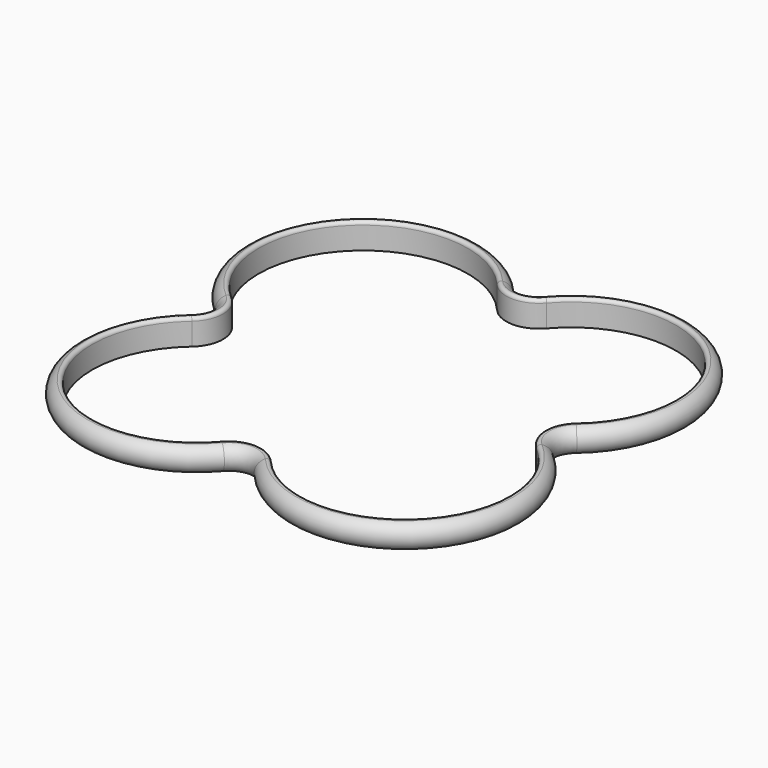
from build123d import *

# Parameters (mm, degrees)
F3_T3_ANGLE  = 98.5086767383
F3_T6_ANGLE  = 188.5086767383
F3_T9_ANGLE  = 98.5086767383
F3_T12_ANGLE = 188.5086767383
F3_T15_ANGLE = 98.5086767383
F3_T18_ANGLE = 188.5086767383
F3_T21_ANGLE = 98.5086767383
F3_T24_ANGLE = 188.5086767383


# Not quite as in the source:
# - a fillet or chamfer that OpenCascade refuses, or shapes differently, is made with other operations: its cross-section is extruded or revolved along the edge and cut away or added


with BuildPart() as f2:
    # F2: sweep along a path in F0
    with BuildLine(Plane.XY) as f2_path:
        ThreePointArc((-7.5761430926, 52.7062817331), (-54.4472211271, 54.4472231756), (-52.706281448, 7.5761450757))
        ThreePointArc((-52.706281448, 7.5761450757), (-49.2333054771, 9.262e-07), (-52.7062817331, -7.5761430926))
        ThreePointArc((-52.7062817331, -7.5761430926), (-54.4472231756, -54.4472211271), (-7.5761450757, -52.706281448))
        ThreePointArc((-7.5761450757, -52.706281448), (-9.262e-07, -49.2333054771), (7.5761430926, -52.7062817331))
        ThreePointArc((7.5761430926, -52.7062817331), (54.4472211271, -54.4472231756), (52.706281448, -7.5761450757))
        ThreePointArc((52.706281448, -7.5761450757), (49.2333054771, -9.262e-07), (52.7062817331, 7.5761430926))
        ThreePointArc((52.7062817331, 7.5761430926), (54.4472231756, 54.4472211271), (7.5761450757, 52.706281448))
        ThreePointArc((7.5761450757, 52.706281448), (9.262e-07, 49.2333054771), (-7.5761430926, 52.7062817331))
    # F1 (on Front) → F2 (sweep)
    with BuildSketch(Plane.XZ):
        with BuildLine():
            ThreePointArc((-49.2333054771, 8), (-53.2333054771, 4), (-49.2333054771, 0))
            Line((-49.2333054771, 0), (-49.2333054771, 8))
        make_face()
    sweep(path=f2_path.line)

    # F3: fillet of radius 1 on 8 edges, made by hand


with BuildPart() as f3_tool1:
    # F3_s2 → F3_t3 (revolve)
    with BuildSketch(Plane(origin=(29.2906767453, 33.9987079499, 0), x_dir=(0, 0, 1), z_dir=(0.6527024029, 0.7576143961, 0))):
        with BuildLine():
            ThreePointArc((7.7712361663, -29.9950533065), (7.6449237057, -29.084369704), (6.8284271247, -28.6617199732))
            Line((6.8284271247, -28.6617199732), (8, -28.6617199732))
            ThreePointArc((8, -28.6617199732), (7.9423942386, -29.3381278881), (7.7712361663, -29.9950533065))
        make_face()
    revolve(axis=Axis((1.1143e-06, 59.2333054771, 8), (0, 0, -1)), revolution_arc=F3_T3_ANGLE)


with BuildPart() as f3_tool4:
    # F3_s5 → F3_t6 (revolve)
    with BuildSketch(Plane(origin=(-29.2906754662, 33.9987090519, 0), x_dir=(0, 0, 1), z_dir=(0.6527023744, -0.7576144207, 0))):
        with BuildLine():
            ThreePointArc((7.7712361663, -29.9950533065), (7.6449237057, -29.084369704), (6.8284271247, -28.6617199732))
            Line((6.8284271247, -28.6617199732), (8, -28.6617199732))
            ThreePointArc((8, -28.6617199732), (7.9423942386, -29.3381278881), (7.7712361663, -29.9950533065))
        make_face()
    revolve(axis=Axis((-31.8198045548, 31.819805752, 8), (0, 0, 1)), revolution_arc=F3_T6_ANGLE)


with BuildPart() as f3_tool7:
    # F3_s8 → F3_t9 (revolve)
    with BuildSketch(Plane(origin=(-33.9987079499, 29.2906767453, 0), x_dir=(0, 0, 1), z_dir=(-0.7576143961, 0.6527024029, 0))):
        with BuildLine():
            ThreePointArc((7.7712361663, -29.9950533065), (7.6449237057, -29.084369704), (6.8284271247, -28.6617199732))
            Line((6.8284271247, -28.6617199732), (8, -28.6617199732))
            ThreePointArc((8, -28.6617199732), (7.9423942386, -29.3381278881), (7.7712361663, -29.9950533065))
        make_face()
    revolve(axis=Axis((-59.2333054771, 1.1143e-06, 8), (0, 0, -1)), revolution_arc=F3_T9_ANGLE)


with BuildPart() as f3_tool10:
    # F3_s11 → F3_t12 (revolve)
    with BuildSketch(Plane(origin=(-33.9987090519, -29.2906754662, 0), x_dir=(0, 0, 1), z_dir=(0.7576144207, 0.6527023744, 0))):
        with BuildLine():
            ThreePointArc((7.7712361663, -29.9950533065), (7.6449237057, -29.084369704), (6.8284271247, -28.6617199732))
            Line((6.8284271247, -28.6617199732), (8, -28.6617199732))
            ThreePointArc((8, -28.6617199732), (7.9423942386, -29.3381278881), (7.7712361663, -29.9950533065))
        make_face()
    revolve(axis=Axis((-31.819805752, -31.8198045548, 8), (0, 0, 1)), revolution_arc=F3_T12_ANGLE)


with BuildPart() as f3_tool13:
    # F3_s14 → F3_t15 (revolve)
    with BuildSketch(Plane(origin=(-29.2906767453, -33.9987079499, 0), x_dir=(0, 0, 1), z_dir=(-0.6527024029, -0.7576143961, 0))):
        with BuildLine():
            ThreePointArc((7.7712361663, -29.9950533065), (7.6449237057, -29.084369704), (6.8284271247, -28.6617199732))
            Line((6.8284271247, -28.6617199732), (8, -28.6617199732))
            ThreePointArc((8, -28.6617199732), (7.9423942386, -29.3381278881), (7.7712361663, -29.9950533065))
        make_face()
    revolve(axis=Axis((-1.1143e-06, -59.2333054771, 8), (0, 0, -1)), revolution_arc=F3_T15_ANGLE)


with BuildPart() as f3_tool16:
    # F3_s17 → F3_t18 (revolve)
    with BuildSketch(Plane(origin=(29.2906754662, -33.9987090519, 0), x_dir=(0, 0, 1), z_dir=(-0.6527023744, 0.7576144207, 0))):
        with BuildLine():
            ThreePointArc((7.7712361663, -29.9950533065), (7.6449237057, -29.084369704), (6.8284271247, -28.6617199732))
            Line((6.8284271247, -28.6617199732), (8, -28.6617199732))
            ThreePointArc((8, -28.6617199732), (7.9423942386, -29.3381278881), (7.7712361663, -29.9950533065))
        make_face()
    revolve(axis=Axis((31.8198045548, -31.819805752, 8), (0, 0, 1)), revolution_arc=F3_T18_ANGLE)


with BuildPart() as f3_tool19:
    # F3_s20 → F3_t21 (revolve)
    with BuildSketch(Plane(origin=(33.9987079499, -29.2906767453, 0), x_dir=(0, 0, 1), z_dir=(0.7576143961, -0.6527024029, 0))):
        with BuildLine():
            ThreePointArc((7.7712361663, -29.9950533065), (7.6449237057, -29.084369704), (6.8284271247, -28.6617199732))
            Line((6.8284271247, -28.6617199732), (8, -28.6617199732))
            ThreePointArc((8, -28.6617199732), (7.9423942386, -29.3381278881), (7.7712361663, -29.9950533065))
        make_face()
    revolve(axis=Axis((59.2333054771, -1.1143e-06, 8), (0, 0, -1)), revolution_arc=F3_T21_ANGLE)


with BuildPart() as f3_tool22:
    # F3_s23 → F3_t24 (revolve)
    with BuildSketch(Plane(origin=(33.9987090519, 29.2906754662, 0), x_dir=(0, 0, 1), z_dir=(-0.7576144207, -0.6527023744, 0))):
        with BuildLine():
            ThreePointArc((7.7712361663, -29.9950533065), (7.6449237057, -29.084369704), (6.8284271247, -28.6617199732))
            Line((6.8284271247, -28.6617199732), (8, -28.6617199732))
            ThreePointArc((8, -28.6617199732), (7.9423942386, -29.3381278881), (7.7712361663, -29.9950533065))
        make_face()
    revolve(axis=Axis((31.819805752, 31.8198045548, 8), (0, 0, 1)), revolution_arc=F3_T24_ANGLE)


with BuildPart() as f2_1:
    add(f2.part)

    # F3_t25: cut F3_tool1, F3_tool4, F3_tool7, F3_tool10, F3_tool13, F3_tool16, F3_tool19, F3_tool22
    add([f3_tool1.part, f3_tool4.part, f3_tool7.part, f3_tool10.part, f3_tool13.part, f3_tool16.part, f3_tool19.part, f3_tool22.part], mode=Mode.SUBTRACT)


solid = f2_1.part
